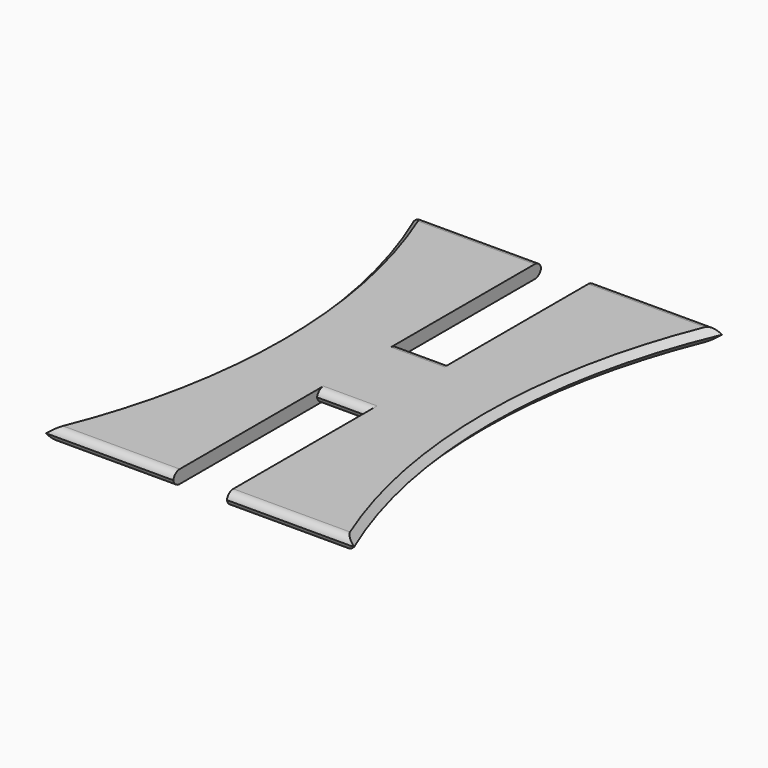
from build123d import *

# Parameters (mm, degrees)
F1_DEPTH    = 2.032
F2_T2_ANGLE = 50.6284103455
F2_T4_ANGLE = 50.6284103455
F2_T6_ANGLE = 50.6284103455
F2_T8_ANGLE = 50.6284103455
F3_T1_DEPTH = 26.2461176682
F3_T3_DEPTH = 24.8658132399
F3_T5_DEPTH = 24.86581324
F3_T7_DEPTH = 26.2461176682
F3_T9_DEPTH = 8.2601420581


# Not quite as in the source:
# - a fillet or chamfer that OpenCascade refuses, or shapes differently, is made with other operations: its cross-section is extruded or revolved along the edge and cut away or added


with BuildPart() as f1:
    # F0 (on Top) → F1 (new body)
    with BuildSketch(Plane.XY):
        with BuildLine():
            Line((-4.1300710291, 54.8246689141), (-24.0261886972, 54.8246689141))
            ThreePointArc((-24.0261886972, 54.8246689141), (-18.5763848247, 37.4605098755), (-16.7346344691, 19.3546451628))
            ThreePointArc((-16.7346344691, 19.3546451628), (-18.5763848247, 1.2487804501), (-24.0261886972, -16.1153785884))
            Line((-24.0261886972, -16.1153785884), (-4.1300710291, -16.1153785884))
            Line((-4.1300710291, -16.1153785884), (-4.1300710291, 11.5803927183))
            Line((-4.1300710291, 11.5803927183), (4.1300710291, 11.5803927183))
            Line((4.1300710291, 11.5803927183), (4.1300710291, -16.1153785884))
            Line((4.1300710291, -16.1153785884), (24.0261886972, -16.1153785884))
            ThreePointArc((24.0261886972, -16.1153785884), (18.5763848247, 1.2487804501), (16.7346344691, 19.3546451628))
            ThreePointArc((16.7346344691, 19.3546451628), (18.5763848247, 37.4605098755), (24.0261886972, 54.8246689141))
            Line((24.0261886972, 54.8246689141), (4.1300710291, 54.8246689141))
            Line((4.1300710291, 54.8246689141), (4.1300710291, 27.1288976073))
            Line((4.1300710291, 27.1288976073), (-4.1300710291, 27.1288976073))
            Line((-4.1300710291, 27.1288976073), (-4.1300710291, 54.8246689141))
        make_face()
    extrude(amount=F1_DEPTH)

    # F2: chamfer of 1.27 on 4 edges, made by hand

    # F2_s1 → F2_t2 (revolve, cut)
    with BuildSketch(Plane(origin=(26.9800180079, 57.0400631379, 0), x_dir=(0, 0, 1), z_dir=(0.4275819968, 0.9039765683, 0))):
        Polygon((2.032, -3.0522508854), (0.762, -1.7822508854), (2.032, -1.7822508854), align=None)
    revolve(axis=Axis((106.6530048847, 19.3546451628, 2.032), (0, 0, 1)), revolution_arc=F2_T2_ANGLE, mode=Mode.SUBTRACT)

    # F2_s3 → F2_t4 (revolve, cut)
    with BuildSketch(Plane(origin=(12.017944167, -25.4078516136, 0), x_dir=(0, 0, 1), z_dir=(0.4275819968, -0.9039765683, 0))):
        Polygon((0, -13.499144765), (1.27, -14.769144765), (0, -14.769144765), align=None)
    revolve(axis=Axis((106.6530048847, 19.3546451628, 0), (0, 0, -1)), revolution_arc=F2_T4_ANGLE, mode=Mode.SUBTRACT)

    # F2_s5 → F2_t6 (revolve, cut)
    with BuildSketch(Plane(origin=(-12.017944167, -25.4078516136, 0), x_dir=(0, 0, 1), z_dir=(-0.4275819968, -0.9039765683, 0))):
        Polygon((2.032, 13.499144765), (0.762, 14.769144765), (2.032, 14.769144765), align=None)
    revolve(axis=Axis((-106.6530048847, 19.3546451628, 2.032), (0, 0, 1)), revolution_arc=F2_T6_ANGLE, mode=Mode.SUBTRACT)

    # F2_s7 → F2_t8 (revolve, cut)
    with BuildSketch(Plane(origin=(-26.9800180079, 57.0400631379, 0), x_dir=(0, 0, 1), z_dir=(-0.4275819968, 0.9039765683, 0))):
        Polygon((1.27, 1.7822508854), (0, 3.0522508854), (0, 1.7822508854), align=None)
    revolve(axis=Axis((-106.6530048847, 19.3546451628, 0), (0, 0, -1)), revolution_arc=F2_T8_ANGLE, mode=Mode.SUBTRACT)

    # F3: fillet of radius 1.27 on 12 edges, made by hand

    # F3_s2 → F3_t1 (cut)
    with BuildSketch(Plane.YZ.offset(-27.2011886972)):
        with BuildLine():
            ThreePointArc((54.8246689141, 1.27), (54.4526945262, 0.3719743879), (53.5546689141, 0))
            Line((53.5546689141, 0), (54.8246689141, 0))
            Line((54.8246689141, 0), (54.8246689141, 1.27))
        make_face()
        with BuildLine():
            ThreePointArc((-16.1153785884, 1.27), (-15.7434042005, 0.3719743879), (-14.8453785884, 0))
            Line((-14.8453785884, 0), (-16.1153785884, 0))
            Line((-16.1153785884, 0), (-16.1153785884, 1.27))
        make_face()
    extrude(amount=F3_T1_DEPTH, mode=Mode.SUBTRACT)

    # F3_s4 → F3_t3 (cut)
    with BuildSketch(Plane.YZ.offset(-25.820884269)):
        with BuildLine():
            ThreePointArc((54.8246689141, 0.762), (54.4526945262, 1.6600256121), (53.5546689141, 2.032))
            Line((53.5546689141, 2.032), (54.8246689141, 2.032))
            Line((54.8246689141, 2.032), (54.8246689141, 0.762))
        make_face()
        with BuildLine():
            ThreePointArc((-16.1153785884, 0.762), (-15.7434042005, 1.6600256121), (-14.8453785884, 2.032))
            Line((-14.8453785884, 2.032), (-16.1153785884, 2.032))
            Line((-16.1153785884, 2.032), (-16.1153785884, 0.762))
        make_face()
    extrude(amount=F3_T3_DEPTH, mode=Mode.SUBTRACT)

    # F3_s6 → F3_t5 (cut)
    with BuildSketch(Plane.YZ.offset(0.9550710291)):
        with BuildLine():
            ThreePointArc((54.8246689141, 0.762), (54.4526945262, 1.6600256121), (53.5546689141, 2.032))
            Line((53.5546689141, 2.032), (54.8246689141, 2.032))
            Line((54.8246689141, 2.032), (54.8246689141, 0.762))
        make_face()
        with BuildLine():
            ThreePointArc((-16.1153785884, 0.762), (-15.7434042005, 1.6600256121), (-14.8453785884, 2.032))
            Line((-14.8453785884, 2.032), (-16.1153785884, 2.032))
            Line((-16.1153785884, 2.032), (-16.1153785884, 0.762))
        make_face()
    extrude(amount=F3_T5_DEPTH, mode=Mode.SUBTRACT)

    # F3_s8 → F3_t7 (cut)
    with BuildSketch(Plane.YZ.offset(0.9550710291)):
        with BuildLine():
            ThreePointArc((54.8246689141, 1.27), (54.4526945262, 0.3719743879), (53.5546689141, 0))
            Line((53.5546689141, 0), (54.8246689141, 0))
            Line((54.8246689141, 0), (54.8246689141, 1.27))
        make_face()
        with BuildLine():
            ThreePointArc((-16.1153785884, 1.27), (-15.7434042005, 0.3719743879), (-14.8453785884, 0))
            Line((-14.8453785884, 0), (-16.1153785884, 0))
            Line((-16.1153785884, 0), (-16.1153785884, 1.27))
        make_face()
    extrude(amount=F3_T7_DEPTH, mode=Mode.SUBTRACT)

    # F3_s10 → F3_t9 (cut)
    with BuildSketch(Plane.YZ.offset(-4.1300710291)):
        with BuildLine():
            ThreePointArc((11.5803927183, 0.762), (11.9523671062, 1.6600256121), (12.8503927183, 2.032))
            Line((12.8503927183, 2.032), (11.5803927183, 2.032))
            Line((11.5803927183, 2.032), (11.5803927183, 0.762))
        make_face()
        with BuildLine():
            ThreePointArc((11.5803927183, 1.27), (11.9523671062, 0.3719743879), (12.8503927183, 0))
            Line((12.8503927183, 0), (11.5803927183, 0))
            Line((11.5803927183, 0), (11.5803927183, 1.27))
        make_face()
        with BuildLine():
            ThreePointArc((27.1288976073, 1.27), (26.7569232194, 0.3719743879), (25.8588976073, 0))
            Line((25.8588976073, 0), (27.1288976073, 0))
            Line((27.1288976073, 0), (27.1288976073, 1.27))
        make_face()
        with BuildLine():
            ThreePointArc((27.1288976073, 0.762), (26.7569232194, 1.6600256121), (25.8588976073, 2.032))
            Line((25.8588976073, 2.032), (27.1288976073, 2.032))
            Line((27.1288976073, 2.032), (27.1288976073, 0.762))
        make_face()
    extrude(amount=F3_T9_DEPTH, mode=Mode.SUBTRACT)


solid = f1.part
